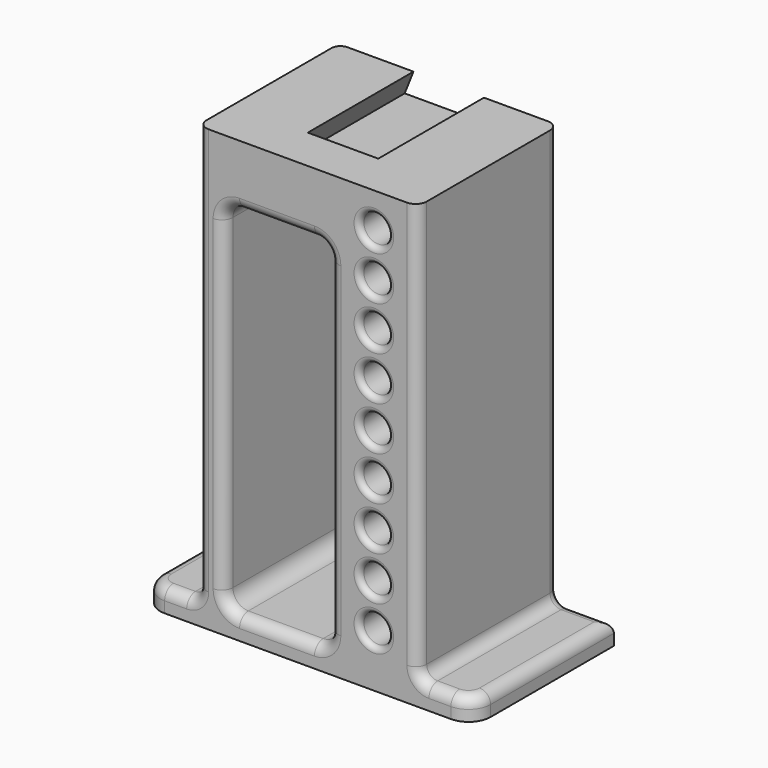
from build123d import *

# Parameters (mm, degrees)
F1_DEPTH     = 20
F2_W         = 75
F2_H         = 40
F3_DEPTH     = 5
F5_DEPTH     = 24
F6_R         = 3.5
F10_R        = 2.5
F11_T1_DEPTH = 5
F11_T4_ANGLE = 90
F11_T6_ANGLE = 90
F13_DEPTH    = 25
F14_R        = 3
F16_R        = 3.25
F17_DEPTH    = 25
F30_R        = 1.25
F31_R        = 2
F33_DEPTH    = 15


# Not quite as in the source:
# - a fillet or chamfer that OpenCascade refuses, or shapes differently, is made with other operations: its cross-section is extruded or revolved along the edge and cut away or added


with BuildPart() as f1:
    # F0 (on Front) → F1 (new body, symmetric)
    with BuildSketch(Plane.XZ):
        Polygon((-25, 0), (0, 0), (25, 0), (25, 100), (-25, 100), align=None)
    extrude(amount=F1_DEPTH, both=True)

    # F2 (on Top) → F3 (join)
    with BuildSketch(Plane.XY):
        Rectangle(F2_W, F2_H)
    extrude(amount=F3_DEPTH)


with BuildPart() as f5:
    # F4 (on Front) → F5 (new body, symmetric)
    with BuildSketch(Plane.XZ):
        Polygon((-19, 5), (0, 5), (5, 5), (5, 86), (-19, 86), align=None)
    extrude(amount=F5_DEPTH, both=True)

    # F6
    f6_edges = [f5.edges().sort_by_distance(p)[0] for p in [
        (-19, 0, 86),
        (5, 0, 86),
        (-19, 0, 5),
        (5, 0, 5),
        (-7, 24, 86),
        (5, 24, 45.5),
        (-19, 24, 45.5),
        (-7, 24, 5),
    ]]
    fillet(f6_edges, radius=F6_R)


with BuildPart() as f5_1:
    # F7: moved
    add(f5.part.moved(Location((0, -8, 0))))


with BuildPart() as f8_1:
    # F8: copy of F5
    add(f5_1.part)


with BuildPart() as f1_1:
    add(f1.part)

    # F9: cut F8_1
    add(f8_1.part, mode=Mode.SUBTRACT)

    # F10
    f10_edges = [f1_1.edges().sort_by_distance(p)[0] for p in [
        (31.25, -20, 5),
        (37.5, 0, 5),
        (25, -20, 52.5),
        (31.25, 20, 5),
        (-31.25, -20, 5),
        (-37.5, 0, 5),
        (-19, -20, 45.5),
        (-25, -20, 52.5),
        (-25, 0, 5),
        (25, 0, 5),
        (-7, -20, 5),
        (3.974874, -20, 6.025126),
        (5, -20, 45.5),
        (3.974874, -20, 84.974874),
        (-7, -20, 86),
        (-17.974874, -20, 84.974874),
        (-17.974874, -20, 6.025126),
        (25, 20, 52.5),
    ]]
    fillet(f10_edges, radius=F10_R)

    # F11: fillet of radius 5 on 2 edges, made by hand

    # F11_s2 → F11_t1 (cut)
    with BuildSketch(Plane.XY):
        with BuildLine():
            ThreePointArc((37.5, -15), (36.0355339059, -18.5355339059), (32.5, -20))
            Line((32.5, -20), (32.5, -20.1))
            Line((32.5, -20.1), (37.6, -20.1))
            Line((37.6, -20.1), (37.6, -15))
            Line((37.6, -15), (37.5, -15))
        make_face()
        with BuildLine():
            ThreePointArc((-32.5, -20), (-36.0355339059, -18.5355339059), (-37.5, -15))
            Line((-37.5, -15), (-37.6, -15))
            Line((-37.6, -15), (-37.6, -20.1))
            Line((-37.6, -20.1), (-32.5, -20.1))
            Line((-32.5, -20.1), (-32.5, -20))
        make_face()
    extrude(amount=F11_T1_DEPTH, mode=Mode.SUBTRACT)

    # F11_s3 → F11_t4 (revolve, cut)
    with BuildSketch(Plane.XZ.offset(15)):
        with BuildLine():
            ThreePointArc((-35, 5), (-36.767766953, 4.267766953), (-37.5, 2.5))
            Line((-37.5, 2.5), (-37.5, 5))
            Line((-37.5, 5), (-35, 5))
        make_face()
    revolve(axis=Axis((-32.5, -15, 5), (0, 0, 1)), revolution_arc=F11_T4_ANGLE, mode=Mode.SUBTRACT)

    # F11_s5 → F11_t6 (revolve, cut)
    with BuildSketch(Plane.YZ.offset(32.5)):
        with BuildLine():
            ThreePointArc((-17.5, 5), (-19.267766953, 4.267766953), (-20, 2.5))
            Line((-20, 2.5), (-20, 5))
            Line((-20, 5), (-17.5, 5))
        make_face()
    revolve(axis=Axis((32.5, -15, 5), (0, 0, 1)), revolution_arc=F11_T6_ANGLE, mode=Mode.SUBTRACT)


with BuildPart() as f13:
    # F12 (on Front) → F13 (new body, symmetric)
    with BuildSketch(Plane.XZ):
        Polygon((-14, 10), (0, 10), (0, 40), (0, 70), (-7, 70), (-14, 70), align=None)
    extrude(amount=F13_DEPTH, both=True)

    # F14
    f14_edges = [f13.edges().sort_by_distance(p)[0] for p in [
        (-14, 0, 70),
        (0, 0, 70),
        (-14, 0, 10),
        (0, 0, 10),
    ]]
    fillet(f14_edges, radius=F14_R)


with BuildPart() as f1_2:
    add(f1_1.part)

    # F15: cut F13
    add(f13.part, mode=Mode.SUBTRACT)


with BuildPart() as f17:
    # F16 (on Front) → F17 (new body)
    with BuildSketch(Plane.XZ):
        with Locations((15, 12)):
            Circle(F16_R)
    extrude(amount=F17_DEPTH)


with BuildPart() as f17_1:
    # F18: moved
    add(f17.part.moved(Location((0, 4, 0))))


with BuildPart() as f19_1:
    # F19: copy of F17
    add(f17_1.part)


with BuildPart() as f20_1:
    # F20: copy of F19_1
    add(f19_1.part)


with BuildPart() as f21_1:
    # F21: copy of F20_1
    add(f20_1.part)


with BuildPart() as f22_1:
    # F22: copy of F21_1
    add(f21_1.part)


with BuildPart() as f19_1_1:
    # F23: moved
    add(f19_1.part.moved(Location((0, 0, 10))))


with BuildPart() as f20_1_1:
    # F24: moved
    add(f20_1.part.moved(Location((0, 0, 20))))


with BuildPart() as f21_1_1:
    # F25: moved
    add(f21_1.part.moved(Location((0, 0, 30))))


with BuildPart() as f22_1_1:
    # F26: moved
    add(f22_1.part.moved(Location((0, 0, 40))))


with BuildPart() as f27_1:
    # F27: copy of F22_1
    add(f22_1_1.part)


with BuildPart() as f27_2:
    # F27: copy of F21_1
    add(f21_1_1.part)


with BuildPart() as f27_3:
    # F27: copy of F20_1
    add(f20_1_1.part)


with BuildPart() as f27_4:
    # F27: copy of F19_1
    add(f19_1_1.part)


with BuildPart() as f27_4_1:
    # F28: moved
    add(f27_4.part.moved(Location((0, 0, 40))))


with BuildPart() as f27_3_1:
    # F28: moved
    add(f27_3.part.moved(Location((0, 0, 40))))


with BuildPart() as f27_2_1:
    # F28: moved
    add(f27_2.part.moved(Location((0, 0, 40))))


with BuildPart() as f27_1_1:
    # F28: moved
    add(f27_1.part.moved(Location((0, 0, 40))))


with BuildPart() as f1_3:
    add(f1_2.part)

    # F29: cut F17, F19_1, F20_1, F21_1, F22_1, F27_4, F27_3, F27_2, F27_1
    add(f17_1.part, mode=Mode.SUBTRACT)
    add(f19_1_1.part, mode=Mode.SUBTRACT)
    add(f20_1_1.part, mode=Mode.SUBTRACT)
    add(f21_1_1.part, mode=Mode.SUBTRACT)
    add(f22_1_1.part, mode=Mode.SUBTRACT)
    add(f27_4_1.part, mode=Mode.SUBTRACT)
    add(f27_3_1.part, mode=Mode.SUBTRACT)
    add(f27_2_1.part, mode=Mode.SUBTRACT)
    add(f27_1_1.part, mode=Mode.SUBTRACT)

    # F30
    f30_edges = [f1_3.edges().sort_by_distance(p)[0] for p in [
        (11.75, -20, 12),
        (11.75, -20, 22),
        (11.75, -20, 32),
        (11.75, -20, 42),
        (11.75, -20, 52),
        (11.75, -20, 62),
        (11.75, -20, 72),
        (11.75, -20, 82),
        (11.75, -20, 92),
    ]]
    fillet(f30_edges, radius=F30_R)

    # F31
    f31_edges = [f1_3.edges().sort_by_distance(p)[0] for p in [
        (-25, 20, 53.75),
        (-7, 16, 70),
        (-37.5, 20, 1.25),
        (-36.767767, 20, 4.267767),
        (-31.25, 20, 5),
        (-25.732233, 20, 5.732233),
    ]]
    fillet(f31_edges, radius=F31_R)


with BuildPart() as f33:
    # F32 (on Front) → F33 (new body, symmetric)
    with BuildSketch(Plane.XZ):
        Polygon((-10, 95), (0, 95), (10, 95), (8, 100), (0, 100), (-8, 100), align=None)
    extrude(amount=F33_DEPTH, both=True)


with BuildPart() as f33_1:
    # F34: moved
    add(f33.part.moved(Location((0, 5, 0))))


with BuildPart() as f1_4:
    add(f1_3.part)

    # F35: cut F33
    add(f33_1.part, mode=Mode.SUBTRACT)


solid = f1_4.part
